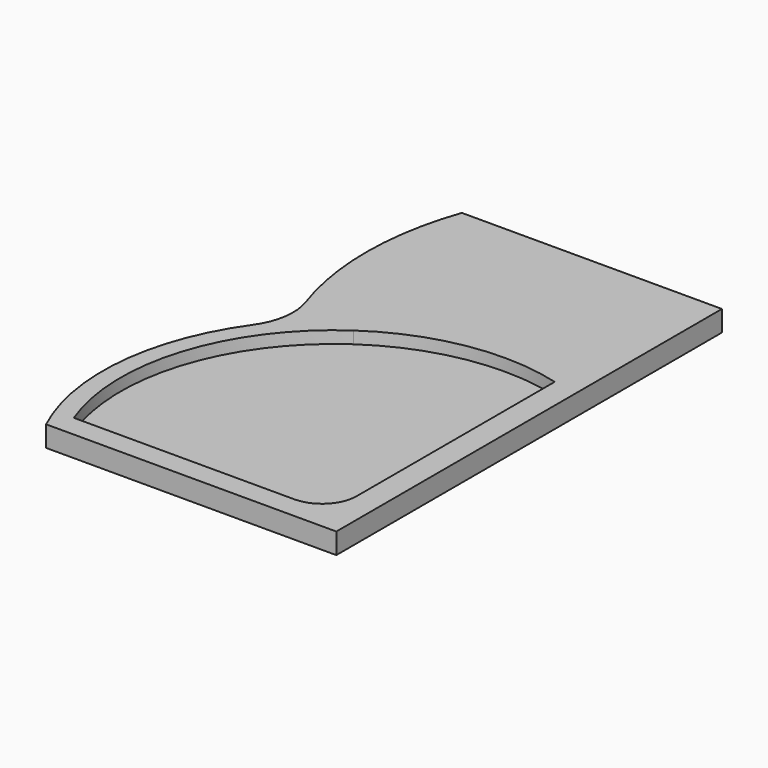
from build123d import *

# Parameters (mm, degrees)
F1_DEPTH = 60
F2_DEPTH = 25


# Not quite as in the source:
# - the program builds the solid bodies; features that only make, move or delete a surface that nothing else refers to are left out


with BuildPart() as f1:
    # F0 (on Top) → F1 (new body)
    with BuildSketch(Plane.XY):
        with BuildLine():
            ThreePointArc((-305.0224336339, -246.0090226419), (-425.7668614501, -572.66743243), (-365.4684518499, -915.6674839367))
            Line((-365.4684518499, -915.6674839367), (-337.7260933976, -915.6674839367))
            ThreePointArc((-337.7260933976, -915.6674839367), (-383.1853890072, -472.5820879471), (-129.4684518499, -106.4961260526))
            ThreePointArc((-129.4684518499, -106.4961260526), (-213.2726615111, 23.7464933662), (-249.4684518499, 174.3325160633))
            Line((-249.4684518499, 174.3325160633), (-249.4684518499, 474.3325160633))
            Line((-249.4684518499, 474.3325160633), (-278.4684518499, 474.3325160633))
            ThreePointArc((-278.4684518499, 474.3325160633), (-327.0089672753, 193.5023169021), (-280.3739250896, -87.6505867625))
            ThreePointArc((-280.3739250896, -87.6505867625), (-274.0048617812, -169.7394217084), (-305.0224336339, -246.0090226419))
        make_face()
        with BuildLine():
            ThreePointArc((-129.4684518499, -106.4961260526), (-383.1853890072, -472.5820879471), (-337.7260933976, -915.6674839367))
            Line((-337.7260933976, -915.6674839367), (-307.8033710716, -915.6674839367))
            ThreePointArc((-307.8033710716, -915.6674839367), (-322.9497717837, -884.2710326331), (-336.294380675, -852.0674300004))
            ThreePointArc((-336.294380675, -852.0674300004), (-349.0076832074, -449.9968879223), (-110.6437650385, -125.9521512216))
            ThreePointArc((-110.6437650385, -125.9521512216), (-120.198249318, -116.3616671102), (-129.4684518499, -106.4961260526))
        make_face()
        with BuildLine():
            ThreePointArc((-336.294380675, -852.0674300004), (-322.9497717837, -884.2710326331), (-307.8033710716, -915.6674839367))
            Line((-307.8033710716, -915.6674839367), (471.5315481501, -915.6674839367))
            Line((471.5315481501, -915.6674839367), (471.5315481501, -255.6674839367))
            Line((471.5315481501, -255.6674839367), (399.6472072601, -255.6674839367))
            Line((399.6472072601, -255.6674839367), (399.6472072601, -752.0674300004))
            ThreePointArc((399.6472072601, -752.0674300004), (370.3578853788, -822.778108119), (299.6472072601, -852.0674300004))
            Line((299.6472072601, -852.0674300004), (-336.294380675, -852.0674300004))
        make_face()
        with BuildLine():
            ThreePointArc((-249.4684518499, 174.3325160633), (-213.2726615111, 23.7464933662), (-129.4684518499, -106.4961260526))
            ThreePointArc((-129.4684518499, -106.4961260526), (-120.198249318, -116.3616671102), (-110.6437650385, -125.9521512216))
            ThreePointArc((-110.6437650385, -125.9521512216), (134.8677667197, -26.0001986196), (399.6472072601, -38.5760851606))
            Line((399.6472072601, -38.5760851606), (399.6472072601, -255.6674839367))
            Line((399.6472072601, -255.6674839367), (471.5315481501, -255.6674839367))
            Line((471.5315481501, -255.6674839367), (471.5315481501, 474.3325160633))
            Line((471.5315481501, 474.3325160633), (-249.4684518499, 474.3325160633))
            Line((-249.4684518499, 474.3325160633), (-249.4684518499, 174.3325160633))
        make_face()
    extrude(amount=F1_DEPTH)

    # F0 (on Top) → F2 (join)
    with BuildSketch(Plane.XY):
        with BuildLine():
            ThreePointArc((-110.6437650385, -125.9521512216), (-349.0076832074, -449.9968879223), (-336.294380675, -852.0674300004))
            Line((-336.294380675, -852.0674300004), (299.6472072601, -852.0674300004))
            ThreePointArc((299.6472072601, -852.0674300004), (370.3578853788, -822.778108119), (399.6472072601, -752.0674300004))
            Line((399.6472072601, -752.0674300004), (399.6472072601, -255.6674839367))
            Line((399.6472072601, -255.6674839367), (171.5315481501, -255.6674839367))
            ThreePointArc((171.5315481501, -255.6674839367), (19.2512340542, -215.1576843257), (-110.6437650385, -125.9521512216))
        make_face()
        with BuildLine():
            ThreePointArc((399.6472072601, -38.5760851606), (134.8677667197, -26.0001986196), (-110.6437650385, -125.9521512216))
            ThreePointArc((-110.6437650385, -125.9521512216), (19.2512340542, -215.1576843257), (171.5315481501, -255.6674839367))
            Line((171.5315481501, -255.6674839367), (399.6472072601, -255.6674839367))
            Line((399.6472072601, -255.6674839367), (399.6472072601, -38.5760851606))
        make_face()
    extrude(amount=F2_DEPTH)


solid = f1.part
